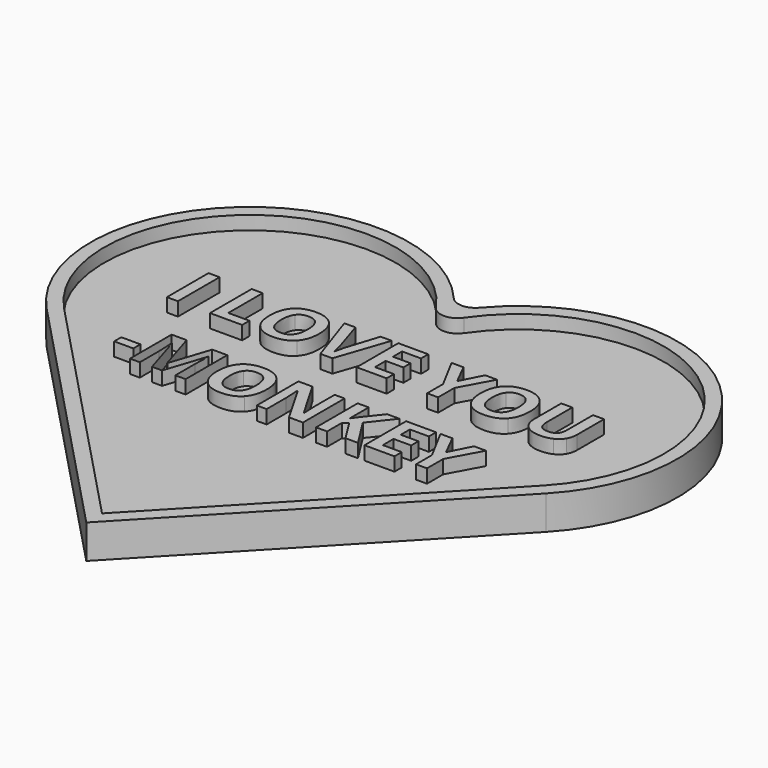
from build123d import *

# Parameters (mm, degrees)
F1_DEPTH = 6.35
F3_W     = 3.5821151422
F3_H     = 1.6672419106
F3_W_2   = 2.0685754307
F3_H_2   = 9.7536853901
F4_DEPTH = 2.54
F5_R     = 3.175


with BuildPart() as f1:
    # F0 (on Top) → F1 (new body)
    with BuildSketch(Plane.XY):
        with BuildLine():
            ThreePointArc((46.753659514, -0.1822602755), (43.5326765205, 43.8575319835), (0, 36.4559032023))
            ThreePointArc((0, 36.4559032023), (-43.5326765205, 43.8575319835), (-46.753659514, -0.1822602755))
            Line((-46.753659514, -0.1822602755), (0, -49.3640825152))
            Line((0, -49.3640825152), (46.753659514, -0.1822602755))
        make_face()
    extrude(amount=F1_DEPTH)

    # F3 (on face) + F2 (on face) → F4 (cut)
    with BuildSketch(Plane.XY.offset(6.35)):
        with BuildLine():
            ThreePointArc((44.9127391314, 1.5677717657), (40.1008944892, 43.1971539593), (0, 31.0284411329))
            ThreePointArc((0, 31.0284411329), (-40.1008944892, 43.1971539593), (-44.9127391314, 1.5677717657))
            Line((-44.9127391314, 1.5677717657), (0, -45.6775214418))
            Line((0, -45.6775214418), (44.9127391314, 1.5677717657))
        make_face()
        with Locations((-30.868062532, -1.1698335161)):
            Rectangle(F3_W, F3_H, mode=Mode.SUBTRACT)
        with BuildLine():
            Line((-21.4196467875, -4.832001887), (-23.3153072441, -4.832001887))
            Line((-23.3153072441, -4.832001887), (-25.6635352873, 2.8189520281))
            Line((-25.6635352873, 2.8189520281), (-25.7233083647, 2.8189520281))
            add(Edge.make_bspline(
                [(-25.7233083647, 2.8189520281), (-25.5952231988, 0.4856672543), (-25.5952231988, -0.2956522582)],
                knots=[0, 0, 0, 1, 1, 1], degree=2))
            Line((-25.5952231988, -0.2956522582), (-25.5952231988, -4.832001887))
            Line((-25.5952231988, -4.832001887), (-27.4439190945, -4.832001887))
            Line((-27.4439190945, -4.832001887), (-27.4439190945, 4.9216835031))
            Line((-27.4439190945, 4.9216835031), (-24.6281801955, 4.9216835031))
            Line((-24.6281801955, 4.9216835031), (-22.3205124549, -2.537142663))
            Line((-22.3205124549, -2.537142663), (-22.2799521524, -2.537142663))
            Line((-22.2799521524, -2.537142663), (-19.8313907292, 4.9216835031))
            Line((-19.8313907292, 4.9216835031), (-17.017786583, 4.9216835031))
            Line((-17.017786583, 4.9216835031), (-17.017786583, -4.832001887))
            Line((-17.017786583, -4.832001887), (-18.9454683311, -4.832001887))
            Line((-18.9454683311, -4.832001887), (-18.9454683311, -0.2145316531))
            add(Edge.make_bspline(
                [(-18.9454683311, -0.2145316531), (-18.9454683311, 0.1120855202), (-18.9347945673, 0.5390360735)],
                knots=[0, 0, 0, 1, 1, 1], degree=2))
            add(Edge.make_bspline(
                [(-18.9347945673, 0.5390360735), (-18.9241208035, 0.9659866268), (-18.8451349511, 2.8061435115)],
                knots=[0, 0, 0, 1, 1, 1], degree=2))
            Line((-18.8451349511, 2.8061435115), (-18.9049080286, 2.8061435115))
            Line((-18.9049080286, 2.8061435115), (-21.4196467875, -4.832001887))
        make_face(mode=Mode.SUBTRACT)
        with BuildLine():
            add(Edge.make_bspline(
                [(-6.9011932226, 3.7806581494), (-5.7100011789, 2.4859305966), (-5.7100011789, 0.058716701)],
                knots=[0, 0, 0, 1, 1, 1], degree=2))
            add(Edge.make_bspline(
                [(-5.7100011789, 0.058716701), (-5.7100011789, -2.3642276889), (-6.91079961, -3.6653595001)],
                knots=[0, 0, 0, 1, 1, 1], degree=2))
            add(Edge.make_bspline(
                [(-6.91079961, -3.6653595001), (-8.1115980412, -4.9664913113), (-10.353088446, -4.9664913113)],
                knots=[0, 0, 0, 1, 1, 1], degree=2))
            add(Edge.make_bspline(
                [(-10.353088446, -4.9664913113), (-12.5945788508, -4.9664913113), (-13.795377282, -3.6653595001)],
                knots=[0, 0, 0, 1, 1, 1], degree=2))
            add(Edge.make_bspline(
                [(-13.795377282, -3.6653595001), (-14.9961757131, -2.3642276889), (-14.9961757131, 0.0715252176)],
                knots=[0, 0, 0, 1, 1, 1], degree=2))
            add(Edge.make_bspline(
                [(-14.9961757131, 0.0715252176), (-14.9961757131, 2.5072781242), (-13.7921751528, 3.7913319133)],
                knots=[0, 0, 0, 1, 1, 1], degree=2))
            add(Edge.make_bspline(
                [(-13.7921751528, 3.7913319133), (-12.5881745925, 5.0753857023), (-10.3402799294, 5.0753857023)],
                knots=[0, 0, 0, 1, 1, 1], degree=2))
            add(Edge.make_bspline(
                [(-10.3402799294, 5.0753857023), (-8.0923852663, 5.0753857023), (-6.9011932226, 3.7806581494)],
                knots=[0, 0, 0, 1, 1, 1], degree=2))
        make_face(mode=Mode.SUBTRACT)
        with BuildLine():
            Line((4.9637626536, 4.9216835031), (4.9637626536, -4.832001887))
            Line((4.9637626536, -4.832001887), (2.3358819981, -4.832001887))
            Line((2.3358819981, -4.832001887), (-1.9080065017, 2.545703674))
            Line((-1.9080065017, 2.545703674), (-1.9677795792, 2.545703674))
            add(Edge.make_bspline(
                [(-1.9677795792, 2.545703674), (-1.8396944132, 0.5924048927), (-1.8396944132, -0.242283439)],
                knots=[0, 0, 0, 1, 1, 1], degree=2))
            Line((-1.8396944132, -0.242283439), (-1.8396944132, -4.832001887))
            Line((-1.8396944132, -4.832001887), (-3.688390309, -4.832001887))
            Line((-3.688390309, -4.832001887), (-3.688390309, 4.9216835031))
            Line((-3.688390309, 4.9216835031), (-1.0797224283, 4.9216835031))
            Line((-1.0797224283, 4.9216835031), (3.1556270604, -2.3834404638))
            Line((3.1556270604, -2.3834404638), (3.2025916213, -2.3834404638))
            add(Edge.make_bspline(
                [(3.2025916213, -2.3834404638), (3.1022582412, -0.4813757489), (3.1022582412, 0.3042132692)],
                knots=[0, 0, 0, 1, 1, 1], degree=2))
            Line((3.1022582412, 0.3042132692), (3.1022582412, 4.9216835031))
            Line((3.1022582412, 4.9216835031), (4.9637626536, 4.9216835031))
        make_face(mode=Mode.SUBTRACT)
        Polygon((11.835531809, 0.6052134093), (15.2639447519, -4.832001887), (12.9157167088, -4.832001887), (10.3604176473, -0.7226028115), (9.4873037658, -1.3502201248), (9.4873037658, -4.832001887), (7.4187283351, -4.832001887), (7.4187283351, 4.9216835031), (9.4873037658, 4.9216835031), (9.4873037658, 0.4579154684), (10.3006445698, 1.6064124568), (12.9434684948, 4.9216835031), (15.2383277187, 4.9216835031), align=None, mode=Mode.SUBTRACT)
        Polygon((22.1079621213, -3.1241996738), (22.1079621213, -4.832001887), (16.4914275927, -4.832001887), (16.4914275927, 4.9216835031), (22.1079621213, 4.9216835031), (22.1079621213, 3.2266898065), (18.5600030234, 3.2266898065), (18.5600030234, 1.0855327817), (21.8624655532, 1.0855327817), (21.8624655532, -0.6094609149), (18.5600030234, -0.6094609149), (18.5600030234, -3.1241996738), align=None, mode=Mode.SUBTRACT)
        Polygon((25.1563890719, 4.9216835031), (27.1779999417, 0.9062135493), (29.2124193282, 4.9216835031), (31.4411012164, 4.9216835031), (28.2048160224, -1.0364114682), (28.2048160224, -4.832001887), (26.1511838611, -4.832001887), (26.1511838611, -1.1025888039), (22.9148986671, 4.9216835031), align=None, mode=Mode.SUBTRACT)
        with Locations((-34.3551811761, 18.6257288876)):
            Rectangle(F3_W_2, F3_H_2, mode=Mode.SUBTRACT)
        Polygon((-21.2915616215, 13.7488861926), (-27.3158339285, 13.7488861926), (-27.3158339285, 23.5025715827), (-25.2472584978, 23.5025715827), (-25.2472584978, 15.4566884058), (-21.2915616215, 15.4566884058), align=None, mode=Mode.SUBTRACT)
        with BuildLine():
            add(Edge.make_bspline(
                [(-11.934940246, 22.361546229), (-10.7437482023, 21.0668186761), (-10.7437482023, 18.6396047806)],
                knots=[0, 0, 0, 1, 1, 1], degree=2))
            add(Edge.make_bspline(
                [(-10.7437482023, 18.6396047806), (-10.7437482023, 16.2166603906), (-11.9445466334, 14.9155285795)],
                knots=[0, 0, 0, 1, 1, 1], degree=2))
            add(Edge.make_bspline(
                [(-11.9445466334, 14.9155285795), (-13.1453450646, 13.6143967683), (-15.3868354694, 13.6143967683)],
                knots=[0, 0, 0, 1, 1, 1], degree=2))
            add(Edge.make_bspline(
                [(-15.3868354694, 13.6143967683), (-17.6283258742, 13.6143967683), (-18.8291243053, 14.9155285795)],
                knots=[0, 0, 0, 1, 1, 1], degree=2))
            add(Edge.make_bspline(
                [(-18.8291243053, 14.9155285795), (-20.0299227365, 16.2166603906), (-20.0299227365, 18.6524132972)],
                knots=[0, 0, 0, 1, 1, 1], degree=2))
            add(Edge.make_bspline(
                [(-20.0299227365, 18.6524132972), (-20.0299227365, 21.0881662038), (-18.8259221762, 22.3722199928)],
                knots=[0, 0, 0, 1, 1, 1], degree=2))
            add(Edge.make_bspline(
                [(-18.8259221762, 22.3722199928), (-17.6219216159, 23.6562737819), (-15.3740269528, 23.6562737819)],
                knots=[0, 0, 0, 1, 1, 1], degree=2))
            add(Edge.make_bspline(
                [(-15.3740269528, 23.6562737819), (-13.1261322897, 23.6562737819), (-11.934940246, 22.361546229)],
                knots=[0, 0, 0, 1, 1, 1], degree=2))
        make_face(mode=Mode.SUBTRACT)
        with BuildLine():
            Line((-5.0055327659, 17.6981788106), (-3.1589716229, 23.5025715827))
            Line((-3.1589716229, 23.5025715827), (-1.0711834173, 23.5025715827))
            Line((-1.0711834173, 23.5025715827), (-4.3864544636, 13.7488861926))
            Line((-4.3864544636, 13.7488861926), (-6.6407533851, 13.7488861926))
            Line((-6.6407533851, 13.7488861926), (-9.9496201731, 23.5025715827))
            Line((-9.9496201731, 23.5025715827), (-7.8618319675, 23.5025715827))
            Line((-7.8618319675, 23.5025715827), (-6.0259445883, 17.6981788106))
            add(Edge.make_bspline(
                [(-6.0259445883, 17.6981788106), (-5.8743771419, 17.1837033939), (-5.7100011789, 16.5005825086)],
                knots=[0, 0, 0, 1, 1, 1], degree=2))
            add(Edge.make_bspline(
                [(-5.7100011789, 16.5005825086), (-5.5456252158, 15.8174616233), (-5.507199666, 15.5506175275)],
                knots=[0, 0, 0, 1, 1, 1], degree=2))
            add(Edge.make_bspline(
                [(-5.507199666, 15.5506175275), (-5.4324833192, 16.1632915715), (-5.0055327659, 17.6981788106)],
                knots=[0, 0, 0, 1, 1, 1], degree=2))
        make_face(mode=Mode.SUBTRACT)
        Polygon((5.7728339521, 15.4566884058), (5.7728339521, 13.7488861926), (0.1562994235, 13.7488861926), (0.1562994235, 23.5025715827), (5.7728339521, 23.5025715827), (5.7728339521, 21.8075778861), (2.2248748542, 21.8075778861), (2.2248748542, 19.6664208613), (5.527337384, 19.6664208613), (5.527337384, 17.9714271647), (2.2248748542, 17.9714271647), (2.2248748542, 15.4566884058), align=None, mode=Mode.SUBTRACT)
        Polygon((12.3713547533, 23.5025715827), (14.3929656232, 19.4871016289), (16.4273850097, 23.5025715827), (18.6560668979, 23.5025715827), (15.4197817039, 17.5444766114), (15.4197817039, 13.7488861926), (13.3661495425, 13.7488861926), (13.3661495425, 17.4782992756), (10.1298643485, 23.5025715827), align=None, mode=Mode.SUBTRACT)
        with BuildLine():
            add(Edge.make_bspline(
                [(27.5451774176, 22.361546229), (28.7363694613, 21.0668186761), (28.7363694613, 18.6396047806)],
                knots=[0, 0, 0, 1, 1, 1], degree=2))
            add(Edge.make_bspline(
                [(28.7363694613, 18.6396047806), (28.7363694613, 16.2166603906), (27.5355710301, 14.9155285795)],
                knots=[0, 0, 0, 1, 1, 1], degree=2))
            add(Edge.make_bspline(
                [(27.5355710301, 14.9155285795), (26.334772599, 13.6143967683), (24.0932821942, 13.6143967683)],
                knots=[0, 0, 0, 1, 1, 1], degree=2))
            add(Edge.make_bspline(
                [(24.0932821942, 13.6143967683), (21.8517917893, 13.6143967683), (20.6509933582, 14.9155285795)],
                knots=[0, 0, 0, 1, 1, 1], degree=2))
            add(Edge.make_bspline(
                [(20.6509933582, 14.9155285795), (19.450194927, 16.2166603906), (19.450194927, 18.6524132972)],
                knots=[0, 0, 0, 1, 1, 1], degree=2))
            add(Edge.make_bspline(
                [(19.450194927, 18.6524132972), (19.450194927, 21.0881662038), (20.6541954873, 22.3722199928)],
                knots=[0, 0, 0, 1, 1, 1], degree=2))
            add(Edge.make_bspline(
                [(20.6541954873, 22.3722199928), (21.8581960476, 23.6562737819), (24.1060907108, 23.6562737819)],
                knots=[0, 0, 0, 1, 1, 1], degree=2))
            add(Edge.make_bspline(
                [(24.1060907108, 23.6562737819), (26.3539853739, 23.6562737819), (27.5451774176, 22.361546229)],
                knots=[0, 0, 0, 1, 1, 1], degree=2))
        make_face(mode=Mode.SUBTRACT)
        with BuildLine():
            Line((36.6349546973, 23.5025715827), (38.6971258697, 23.5025715827))
            Line((38.6971258697, 23.5025715827), (38.6971258697, 17.1922424049))
            add(Edge.make_bspline(
                [(38.6971258697, 17.1922424049), (38.6971258697, 16.1099227523), (38.2136043681, 15.2965819483)],
                knots=[0, 0, 0, 1, 1, 1], degree=2))
            add(Edge.make_bspline(
                [(38.2136043681, 15.2965819483), (37.7300828665, 14.4832411442), (36.8153413061, 14.0488189563)],
                knots=[0, 0, 0, 1, 1, 1], degree=2))
            add(Edge.make_bspline(
                [(36.8153413061, 14.0488189563), (35.9005997456, 13.6143967683), (34.65390413, 13.6143967683)],
                knots=[0, 0, 0, 1, 1, 1], degree=2))
            add(Edge.make_bspline(
                [(34.65390413, 13.6143967683), (32.7731869427, 13.6143967683), (31.7324949691, 14.5793050187)],
                knots=[0, 0, 0, 1, 1, 1], degree=2))
            add(Edge.make_bspline(
                [(31.7324949691, 14.5793050187), (30.6918029954, 15.5442132692), (30.6918029954, 17.2178594381)],
                knots=[0, 0, 0, 1, 1, 1], degree=2))
            Line((30.6918029954, 17.2178594381), (30.6918029954, 23.5025715827))
            Line((30.6918029954, 23.5025715827), (32.7518394151, 23.5025715827))
            Line((32.7518394151, 23.5025715827), (32.7518394151, 17.5316680948))
            add(Edge.make_bspline(
                [(32.7518394151, 17.5316680948), (32.7518394151, 16.4045186341), (33.2054743779, 15.8772347008)],
                knots=[0, 0, 0, 1, 1, 1], degree=2))
            add(Edge.make_bspline(
                [(33.2054743779, 15.8772347008), (33.6591093408, 15.3499507674), (34.7072729492, 15.3499507674)],
                knots=[0, 0, 0, 1, 1, 1], degree=2))
            add(Edge.make_bspline(
                [(34.7072729492, 15.3499507674), (35.7212805133, 15.3499507674), (36.1781176053, 15.8804368299)],
                knots=[0, 0, 0, 1, 1, 1], degree=2))
            add(Edge.make_bspline(
                [(36.1781176053, 15.8804368299), (36.6349546973, 16.4109228924), (36.6349546973, 17.5444766114)],
                knots=[0, 0, 0, 1, 1, 1], degree=2))
            Line((36.6349546973, 17.5444766114), (36.6349546973, 23.5025715827))
        make_face(mode=Mode.SUBTRACT)
        with BuildLine():
            add(Edge.make_bspline(
                [(-17.2344639888, 21.1031094731), (-17.8610139257, 20.272690647), (-17.8610139257, 18.6396047806)],
                knots=[0, 0, 0, 1, 1, 1], degree=2))
            add(Edge.make_bspline(
                [(-17.8610139257, 18.6396047806), (-17.8610139257, 17.0043841615), (-17.2408682471, 16.1771674645)],
                knots=[0, 0, 0, 1, 1, 1], degree=2))
            add(Edge.make_bspline(
                [(-17.2408682471, 16.1771674645), (-16.6207225684, 15.3499507674), (-15.3868354694, 15.3499507674)],
                knots=[0, 0, 0, 1, 1, 1], degree=2))
            add(Edge.make_bspline(
                [(-15.3868354694, 15.3499507674), (-12.912657013, 15.3499507674), (-12.912657013, 18.6396047806)],
                knots=[0, 0, 0, 1, 1, 1], degree=2))
            add(Edge.make_bspline(
                [(-12.912657013, 18.6396047806), (-12.912657013, 21.9335282993), (-15.3740269528, 21.9335282993)],
                knots=[0, 0, 0, 1, 1, 1], degree=2))
            add(Edge.make_bspline(
                [(-15.3740269528, 21.9335282993), (-16.6079140518, 21.9335282993), (-17.2344639888, 21.1031094731)],
                knots=[0, 0, 0, 1, 1, 1], degree=2))
        make_face()
        with BuildLine():
            add(Edge.make_bspline(
                [(22.2456536748, 21.1031094731), (21.6191037378, 20.272690647), (21.6191037378, 18.6396047806)],
                knots=[0, 0, 0, 1, 1, 1], degree=2))
            add(Edge.make_bspline(
                [(21.6191037378, 18.6396047806), (21.6191037378, 17.0043841615), (22.2392494165, 16.1771674645)],
                knots=[0, 0, 0, 1, 1, 1], degree=2))
            add(Edge.make_bspline(
                [(22.2392494165, 16.1771674645), (22.8593950951, 15.3499507674), (24.0932821942, 15.3499507674)],
                knots=[0, 0, 0, 1, 1, 1], degree=2))
            add(Edge.make_bspline(
                [(24.0932821942, 15.3499507674), (26.5674606505, 15.3499507674), (26.5674606505, 18.6396047806)],
                knots=[0, 0, 0, 1, 1, 1], degree=2))
            add(Edge.make_bspline(
                [(26.5674606505, 18.6396047806), (26.5674606505, 21.9335282993), (24.1060907108, 21.9335282993)],
                knots=[0, 0, 0, 1, 1, 1], degree=2))
            add(Edge.make_bspline(
                [(24.1060907108, 21.9335282993), (22.8722036117, 21.9335282993), (22.2456536748, 21.1031094731)],
                knots=[0, 0, 0, 1, 1, 1], degree=2))
        make_face()
    with BuildSketch(Plane.XY.offset(6.35)):
        with BuildLine():
            add(Edge.make_bspline(
                [(-12.0418901448, 2.497742511), (-12.6684400818, 1.6673236849), (-12.6684400818, 0.0342378185)],
                knots=[0, 0, 0, 1, 1, 1], degree=2))
            add(Edge.make_bspline(
                [(-12.6684400818, 0.0342378185), (-12.6684400818, -1.6009828006), (-12.0482944031, -2.4281994977)],
                knots=[0, 0, 0, 1, 1, 1], degree=2))
            add(Edge.make_bspline(
                [(-12.0482944031, -2.4281994977), (-11.4281487245, -3.2554161947), (-10.1942616254, -3.2554161947)],
                knots=[0, 0, 0, 1, 1, 1], degree=2))
            add(Edge.make_bspline(
                [(-10.1942616254, -3.2554161947), (-7.7200831691, -3.2554161947), (-7.7200831691, 0.0342378185)],
                knots=[0, 0, 0, 1, 1, 1], degree=2))
            add(Edge.make_bspline(
                [(-7.7200831691, 0.0342378185), (-7.7200831691, 3.3281613372), (-10.1814531088, 3.3281613372)],
                knots=[0, 0, 0, 1, 1, 1], degree=2))
            add(Edge.make_bspline(
                [(-10.1814531088, 3.3281613372), (-11.4153402079, 3.3281613372), (-12.0418901448, 2.497742511)],
                knots=[0, 0, 0, 1, 1, 1], degree=2))
        make_face()
    extrude(amount=-F4_DEPTH, mode=Mode.SUBTRACT)

    # F5
    f5_edges = [f1.edges().sort_by_distance(p)[0] for p in [
        (0, 36.455903, 3.175),
        (0, 31.028441, 5.08),
    ]]
    fillet(f5_edges, radius=F5_R)


solid = f1.part
